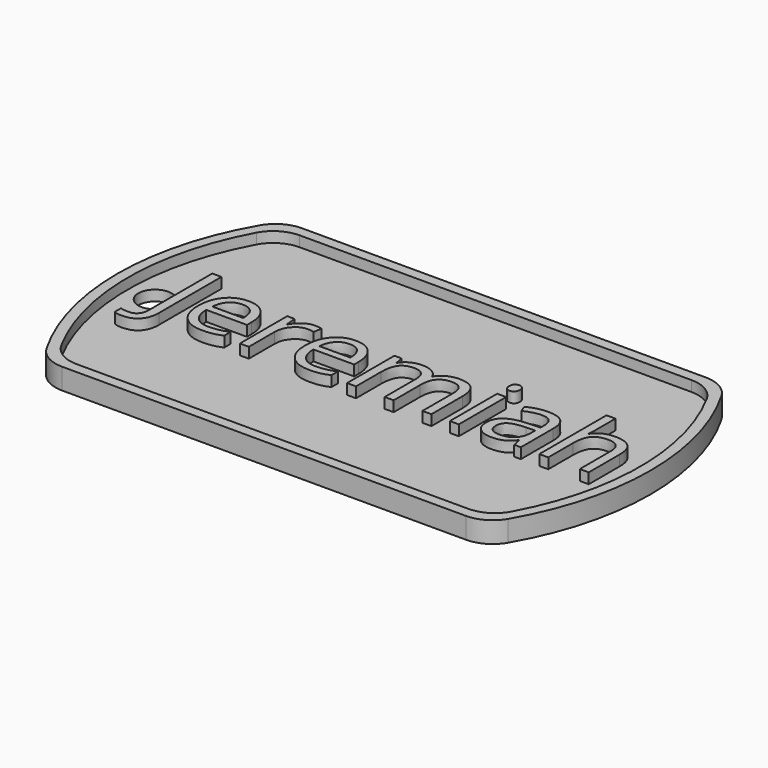
from build123d import *

# Parameters (mm, degrees)
F1_DEPTH     = 1
F3_DEPTH     = 1
F4_R         = 1.5875
F5_DEPTH     = 1
F6_TEXT_SIZE = 10.533256702
F7_DEPTH     = 1


# Not quite as in the source:
# - Text() gives the source's letters only with a copy of the font that has no kerning and outlines rounded to 1/6400 em; it was checked with that copy


with BuildPart() as f1:
    # F0 (on Top) → F1 (new body)
    with BuildSketch(Plane.XY):
        with BuildLine():
            ThreePointArc((-19.2474145991, 14.2875), (-20.8349145991, 13.862130657), (-21.9970452561, 12.7))
            ThreePointArc((-21.9970452561, 12.7), (-25.4, 0), (-21.9970452561, -12.7))
            ThreePointArc((-21.9970452561, -12.7), (-20.8349145991, -13.862130657), (-19.2474145991, -14.2875))
            Line((-19.2474145991, -14.2875), (19.2474145991, -14.2875))
            ThreePointArc((19.2474145991, -14.2875), (20.8349145991, -13.862130657), (21.9970452561, -12.7))
            ThreePointArc((21.9970452561, -12.7), (25.4, 0), (21.9970452561, 12.7))
            ThreePointArc((21.9970452561, 12.7), (20.8349145991, 13.862130657), (19.2474145991, 14.2875))
            Line((19.2474145991, 14.2875), (-19.2474145991, 14.2875))
        make_face()
    extrude(amount=F1_DEPTH)

    # F2 (on face) → F3 (join)
    with BuildSketch(Plane.XY.offset(1)):
        with BuildLine():
            Line((19.2474145991, 14.2875), (-19.2474145991, 14.2875))
            ThreePointArc((-19.2474145991, 14.2875), (-20.8349145991, 13.862130657), (-21.9970452561, 12.7))
            ThreePointArc((-21.9970452561, 12.7), (-25.4, 0), (-21.9970452561, -12.7))
            ThreePointArc((-21.9970452561, -12.7), (-20.8349145991, -13.862130657), (-19.2474145991, -14.2875))
            Line((-19.2474145991, -14.2875), (19.2474145991, -14.2875))
            ThreePointArc((19.2474145991, -14.2875), (20.8349145991, -13.862130657), (21.9970452561, -12.7))
            ThreePointArc((21.9970452561, -12.7), (25.4, 0), (21.9970452561, 12.7))
            ThreePointArc((21.9970452561, 12.7), (20.8349145991, 13.862130657), (19.2474145991, 14.2875))
        make_face()
        with BuildLine():
            ThreePointArc((-21.4526124879, 11.6252061249), (-20.2856017842, 12.8404540819), (-18.6611352482, 13.2875))
            Line((-18.6611352482, 13.2875), (18.6611352482, 13.2875))
            ThreePointArc((18.6611352482, 13.2875), (20.2856017842, 12.8404540819), (21.4526124879, 11.6252061249))
            ThreePointArc((21.4526124879, 11.6252061249), (24.4, 0), (21.4526124879, -11.6252061249))
            ThreePointArc((21.4526124879, -11.6252061249), (20.2856017842, -12.8404540819), (18.6611352482, -13.2875))
            Line((18.6611352482, -13.2875), (-18.6611352482, -13.2875))
            ThreePointArc((-18.6611352482, -13.2875), (-20.2856017842, -12.8404540819), (-21.4526124879, -11.6252061249))
            ThreePointArc((-21.4526124879, -11.6252061249), (-24.4, 0), (-21.4526124879, 11.6252061249))
        make_face(mode=Mode.SUBTRACT)
    extrude(amount=F3_DEPTH)

    # F4 (on face) → F5 (cut)
    with BuildSketch(Plane.XY.offset(1)):
        with Locations((-21.821282804, 0)):
            Circle(F4_R)
    extrude(amount=-F5_DEPTH, mode=Mode.SUBTRACT)

    # F6 (on face) → F7 (join)
    with BuildSketch(Plane.XY.offset(1)):
        with Locations((-20.8809208125, -3.0985514168)):
            Text('Jeremiah', F6_TEXT_SIZE, font='Open Sans', text_align=(TextAlign.LEFT, TextAlign.BOTTOM))
    extrude(amount=F7_DEPTH)


solid = f1.part
